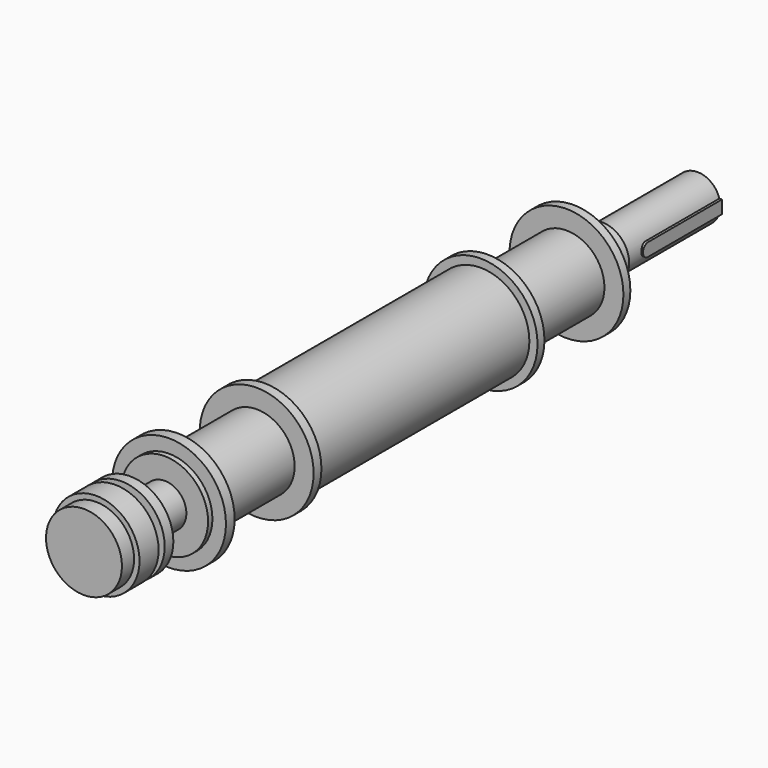
from build123d import *

# Parameters (mm, degrees)
F0_R      = 21
F1_DEPTH  = 110
F3_DEPTH  = 22.5
F4_R      = 25
F5_DEPTH  = 23
F6_R      = 37.5
F7_DEPTH  = 10
F8_R      = 9.99999
F9_R      = 52.5
F9_R_2    = 37.5
F10_DEPTH = 8
F11_R     = 35
F12_DEPTH = 91
F13_R     = 52.5
F14_DEPTH = 8
F15_R     = 45
F16_DEPTH = 249
F17_R     = 52.5
F18_DEPTH = 9
F19_R     = 35
F20_DEPTH = 91
F21_R     = 52.5
F22_DEPTH = 10
F23_R     = 40
F24_DEPTH = 5
F25_R     = 20
F26_DEPTH = 40
F27_R     = 40
F28_DEPTH = 10
F29_R     = 30
F30_DEPTH = 7
F31_R     = 40
F32_DEPTH = 22
F33_R     = 35
F34_DEPTH = 14


# Not quite as in the source:
# - a fillet or chamfer is up to 0.001 mm smaller than in the source, because OpenCascade refuses the exact size


with BuildPart() as f1:
    # F0 (on Front) → F1 (new body)
    with BuildSketch(Plane.XZ):
        Circle(F0_R)
    extrude(amount=F1_DEPTH)

    # F2 (on Right) → F3 (join)
    with BuildSketch(Plane.YZ):
        with BuildLine():
            Line((0, -6), (0, 6))
            Line((0, 6), (-85, 6))
            ThreePointArc((-85, 6), (-91, 0), (-85, -6))
            Line((-85, -6), (0, -6))
        make_face()
    extrude(amount=F3_DEPTH)

    # F4 (on face) → F5 (join)
    with BuildSketch(Plane.XZ.offset(110)):
        Circle(F4_R)
    extrude(amount=F5_DEPTH)

    # F6 (on face) → F7 (join)
    with BuildSketch(Plane.XZ.offset(133)):
        Circle(F6_R)
    extrude(amount=F7_DEPTH)

    # F8 (radius 10 in the source; OpenCascade refuses exactly that, so slightly less here)
    f8_edges = [f1.edges().sort_by_distance(p)[0] for p in [
        (-37.5, -133, 0),
    ]]
    fillet(f8_edges, radius=F8_R)

    # F9 (on face) → F10 (join)
    with BuildSketch(Plane.XZ.offset(143)):
        Circle(F9_R)
        Circle(F9_R_2, mode=Mode.SUBTRACT)
        Circle(F9_R_2)
    extrude(amount=F10_DEPTH)

    # F11 (on face) → F12 (join)
    with BuildSketch(Plane.XZ.offset(151)):
        Circle(F11_R)
    extrude(amount=F12_DEPTH)

    # F13 (on face) → F14 (join)
    with BuildSketch(Plane.XZ.offset(242)):
        Circle(F13_R)
    extrude(amount=F14_DEPTH)

    # F15 (on face) → F16 (join)
    with BuildSketch(Plane.XZ.offset(250)):
        Circle(F15_R)
    extrude(amount=F16_DEPTH)

    # F17 (on face) → F18 (join)
    with BuildSketch(Plane.XZ.offset(499)):
        Circle(F17_R)
    extrude(amount=F18_DEPTH)

    # F19 (on face) → F20 (join)
    with BuildSketch(Plane.XZ.offset(508)):
        Circle(F19_R)
    extrude(amount=F20_DEPTH)

    # F21 (on face) → F22 (join)
    with BuildSketch(Plane.XZ.offset(599)):
        Circle(F21_R)
    extrude(amount=F22_DEPTH)

    # F23 (on face) → F24 (join)
    with BuildSketch(Plane.XZ.offset(609)):
        Circle(F23_R)
    extrude(amount=F24_DEPTH)

    # F25 (on face) → F26 (join)
    with BuildSketch(Plane.XZ.offset(614)):
        Circle(F25_R)
    extrude(amount=F26_DEPTH)

    # F27 (on face) → F28 (join)
    with BuildSketch(Plane.XZ.offset(654)):
        Circle(F27_R)
    extrude(amount=F28_DEPTH)

    # F29 (on face) → F30 (join)
    with BuildSketch(Plane.XZ.offset(664)):
        Circle(F29_R)
    extrude(amount=F30_DEPTH)

    # F31 (on face) → F32 (join)
    with BuildSketch(Plane.XZ.offset(671)):
        Circle(F31_R)
    extrude(amount=F32_DEPTH)

    # F33 (on face) → F34 (join)
    with BuildSketch(Plane.XZ.offset(693)):
        Circle(F33_R)
    extrude(amount=F34_DEPTH)


solid = f1.part
